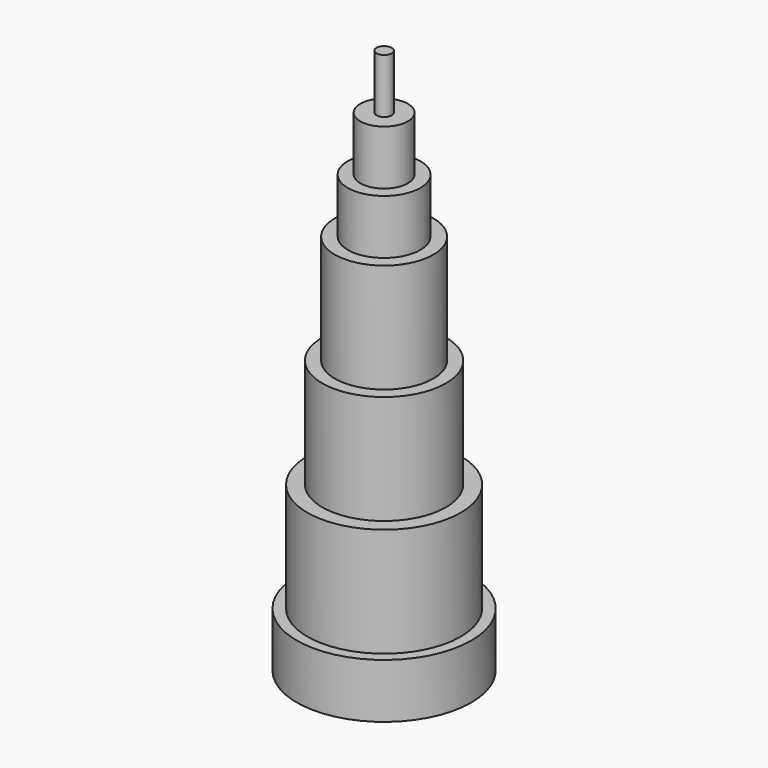
from build123d import *

# Parameters (mm, degrees)
F0_R     = 3.522094475
F1_DEPTH = 254
F0_R_2   = 40.599940794
F0_R_3   = 35.6715893611
F2_DEPTH = 25.4
F0_R_4   = 28.8071763317
F3_DEPTH = 76.2
F0_R_5   = 22.9201353623
F4_DEPTH = 127
F0_R_6   = 16.8984108621
F5_DEPTH = 177.8
F0_R_7   = 11.0751082581
F6_DEPTH = 203.2
F7_DEPTH = 228.6


# Not quite as in the source:
# - the program builds the solid bodies; features that only make, move or delete a surface that nothing else refers to are left out


with BuildPart() as f1:
    # F0 (on Top) → F1 (new body)
    with BuildSketch(Plane.XY):
        Circle(F0_R)
    extrude(amount=F1_DEPTH)


with BuildPart() as f2:
    # F0 (on Top) → F2 (new body)
    with BuildSketch(Plane.XY):
        Circle(F0_R_2)
        Circle(F0_R_3, mode=Mode.SUBTRACT)
    extrude(amount=F2_DEPTH)

    # F0 (on Top) → F3 (join)
    with BuildSketch(Plane.XY):
        Circle(F0_R_3)
        Circle(F0_R_4, mode=Mode.SUBTRACT)
    extrude(amount=F3_DEPTH)

    # F0 (on Top) → F4 (join)
    with BuildSketch(Plane.XY):
        Circle(F0_R_4)
        Circle(F0_R_5, mode=Mode.SUBTRACT)
    extrude(amount=F4_DEPTH)

    # F0 (on Top) → F5 (join)
    with BuildSketch(Plane.XY):
        Circle(F0_R_5)
        Circle(F0_R_6, mode=Mode.SUBTRACT)
    extrude(amount=F5_DEPTH)

    # F0 (on Top) → F6 (join)
    with BuildSketch(Plane.XY):
        Circle(F0_R_6)
        Circle(F0_R_7, mode=Mode.SUBTRACT)
    extrude(amount=F6_DEPTH)


with BuildPart() as f7:
    # F0 (on Top) → F7 (new body)
    with BuildSketch(Plane.XY):
        Circle(F0_R_7)
        Circle(F0_R, mode=Mode.SUBTRACT)
    extrude(amount=F7_DEPTH)


solid = Compound([f1.part, f2.part, f7.part])
